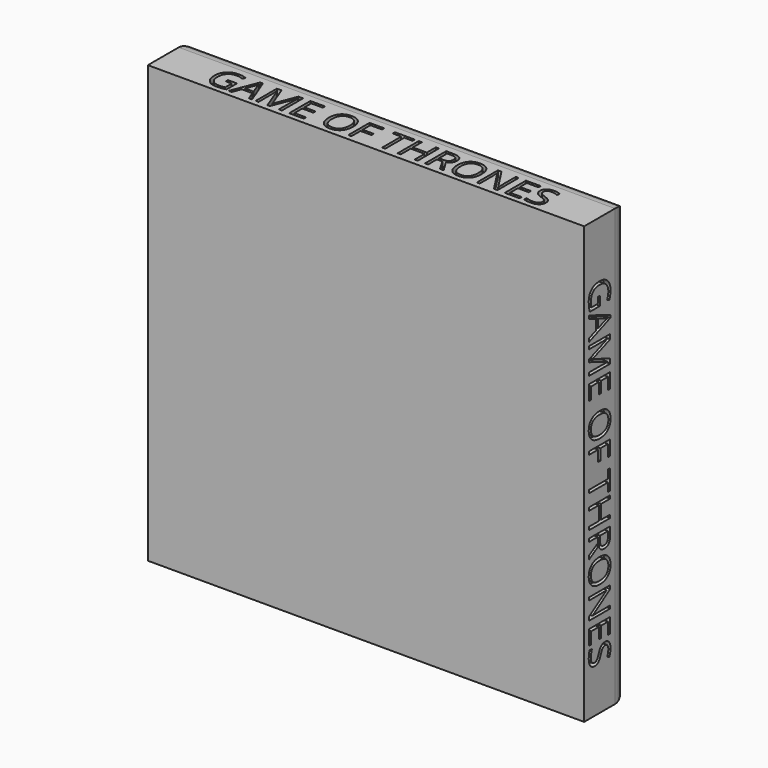
from build123d import *

# Parameters (mm, degrees)
F1_W          = 146.05
F1_H          = 146.05
F2_DEPTH      = 19.05
F0_W          = 127.762
F0_H          = 127.762
F3_DEPTH      = 6.858
F4_R          = 6.1321024484
F5_TEXT_SIZE  = 12.4157186494
F6_DEPTH      = 2.032
F7_TEXT_SIZE  = 12.4157186494
F8_DEPTH      = 2.032
F9_TEXT_SIZE  = 12.0888069634
F10_DEPTH     = 2.032
F11_TEXT_SIZE = 11.5927567499
F12_DEPTH     = 2.032


# Not quite as in the source:
# - Text() gives the source's letters only with a copy of the font that has no kerning and outlines rounded to 1/6400 em; it was checked with that copy


with BuildPart() as f2:
    # F1 (on Front) → F2 (new body)
    with BuildSketch(Plane.XZ):
        Rectangle(F1_W, F1_H)
    extrude(amount=F2_DEPTH)

    # F0 (on Front) → F3 (cut)
    with BuildSketch(Plane.XZ):
        Rectangle(F0_W, F0_H)
    extrude(amount=F3_DEPTH, mode=Mode.SUBTRACT)

    # F4
    f4_edges = [f2.edges().sort_by_distance(p)[0] for p in [
        (73.025, 0, 0),
        (0, 0, -73.025),
        (-73.025, 0, 0),
        (0, 0, 73.025),
    ]]
    fillet(f4_edges, radius=F4_R)

    # F5 (on face) → F6 (cut)
    with BuildSketch(Plane.XY.offset(73.025)):
        with Locations((-56.500710547, -17.2228384763)):
            Text('GAME OF THRONES', F5_TEXT_SIZE, font='Open Sans', text_align=(TextAlign.LEFT, TextAlign.BOTTOM))
    extrude(amount=-F6_DEPTH, mode=Mode.SUBTRACT)

    # F7 (on face) → F8 (cut)
    with BuildSketch(Plane.YZ.offset(73.025)):
        with Locations(Location((-17.0166593173, 54.9926923693), (0, 0, -90))):
            Text('GAME OF THRONES', F7_TEXT_SIZE, font='Open Sans', text_align=(TextAlign.LEFT, TextAlign.BOTTOM))
    extrude(amount=-F8_DEPTH, mode=Mode.SUBTRACT)

    # F9 (on face) → F10 (cut)
    with BuildSketch(Plane(origin=(0, 0, -73.025), x_dir=(1, 0, 0), z_dir=(0, 0, -1))):
        with Locations(Location((54.7907940386, 16.9010008685), (0, 0, -180))):
            Text('GAME OF THRONES', F9_TEXT_SIZE, font='Open Sans', text_align=(TextAlign.LEFT, TextAlign.BOTTOM))
    extrude(amount=-F10_DEPTH, mode=Mode.SUBTRACT)

    # F11 (on face) → F12 (cut)
    with BuildSketch(Plane(origin=(-73.025, 0, 0), x_dir=(0, -1, 0), z_dir=(-1, 0, 0))):
        with Locations(Location((16.3413972182, -55.1973950638), (0, 0, 90))):
            Text('GAME OF THRONES', F11_TEXT_SIZE, font='Open Sans', text_align=(TextAlign.LEFT, TextAlign.BOTTOM))
    extrude(amount=-F12_DEPTH, mode=Mode.SUBTRACT)


solid = f2.part
